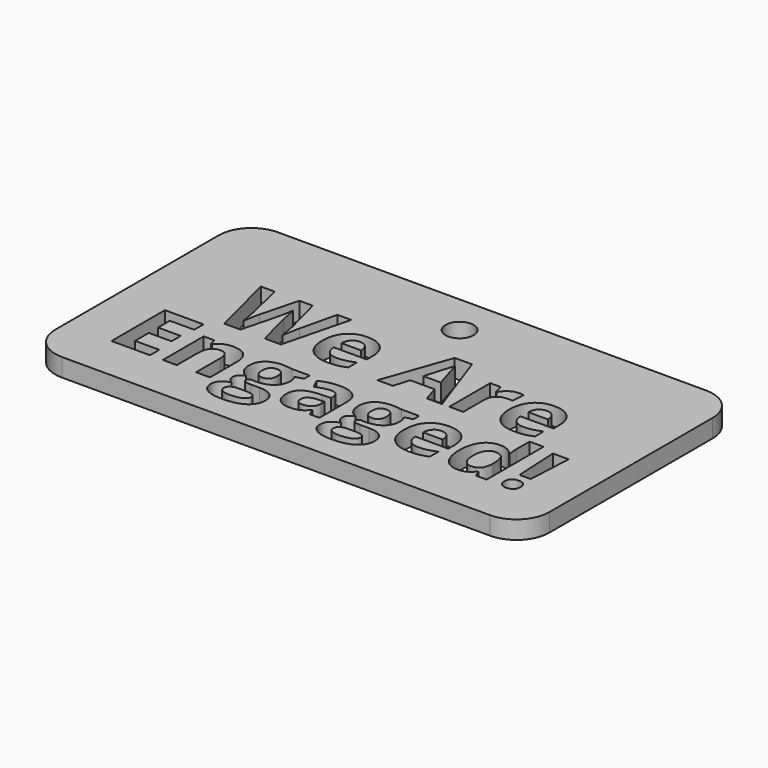
from build123d import *

# Parameters (mm, degrees)
F1_W          = 152.6316851377
F1_H          = 83.4434144199
F2_DEPTH      = 5.588
F0_R          = 4.3339289333
F0_TEXT_SIZE  = 28.9214568006
F3_DEPTH      = 38.862
F3_DEPTH_BACK = 25.4
F4_R          = 10.16
F5_R          = 10.16
F6_R          = 10.16


# Not quite as in the source:
# - Text() gives the source's letters only with a copy of the font that has no kerning and outlines rounded to 1/6400 em; it was checked with that copy


with BuildPart() as f2:
    # F1 (on Top) → F2 (new body)
    with BuildSketch(Plane.XY):
        with Locations((0.0068917871, -2.6251468807)):
            Rectangle(F1_W, F1_H)
    extrude(amount=F2_DEPTH)

    # F0 (on Top) → F3 (cut, two sides)
    with BuildSketch(Plane.XY) as f3_sk:
        with Locations((0, 26.5802778304)):
            Circle(F0_R)
        with Locations((-51.685806587, -6.2457583845)):
            Text('We Are', F0_TEXT_SIZE, font='Open Sans', font_style=FontStyle.BOLD, text_align=(TextAlign.LEFT, TextAlign.BOTTOM))
        with Locations((-64.6055636171, -30.3413132206)):
            Text('Engaged!', F0_TEXT_SIZE, font='Open Sans', font_style=FontStyle.BOLD, text_align=(TextAlign.LEFT, TextAlign.BOTTOM))
    extrude(amount=-F3_DEPTH, mode=Mode.SUBTRACT)
    extrude(f3_sk.sketch, amount=F3_DEPTH_BACK, mode=Mode.SUBTRACT)

    # F4
    f4_edges = [f2.edges().sort_by_distance(p)[0] for p in [
        (-76.308951, -44.346854, 2.794),
    ]]
    fillet(f4_edges, radius=F4_R)

    # F5
    f5_edges = [f2.edges().sort_by_distance(p)[0] for p in [
        (-76.308951, 39.09656, 2.794),
    ]]
    fillet(f5_edges, radius=F5_R)

    # F6
    f6_edges = [f2.edges().sort_by_distance(p)[0] for p in [
        (76.322734, 39.09656, 2.794),
        (76.322734, -44.346854, 2.794),
    ]]
    fillet(f6_edges, radius=F6_R)


solid = f2.part
